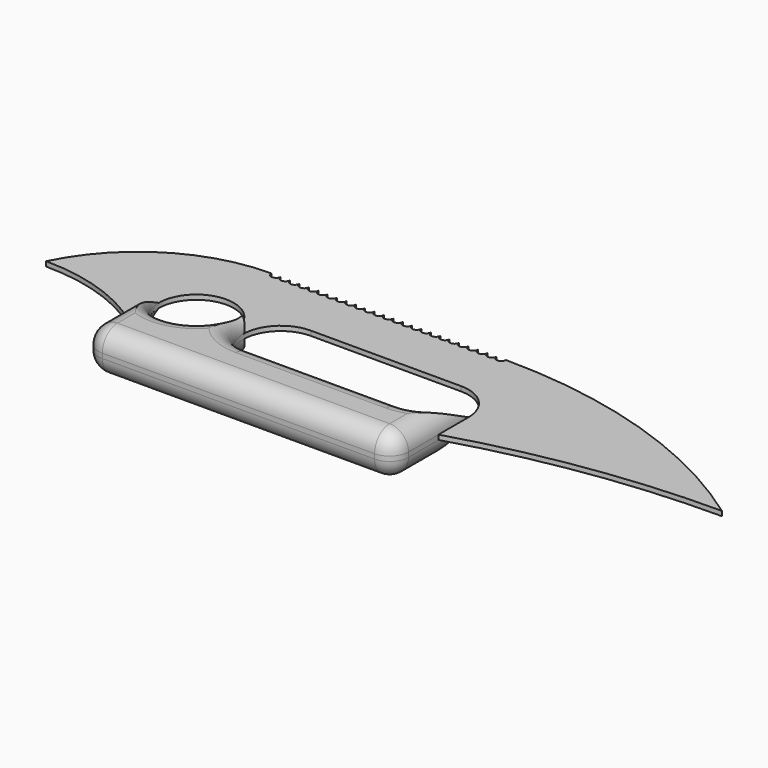
from build123d import *

# Parameters (mm, degrees)
F0_R           = 12.7
F1_DEPTH       = 1.5875
F3_DEPTH       = 6.35
F5_DEPTH       = 6.35
F6_T1_DEPTH    = 92.075
F6_T3_DEPTH    = 41.275
F6_T5_DEPTH    = 50.8
F6_T8_ANGLE    = 323.4698049006
F6_T10_ANGLE   = 90
F6_T12_ANGLE   = 90
F6_T14_ANGLE   = 161.6484946187
F6_T16_ANGLE   = 161.6484946187
F6_2_T1_DEPTH  = 92.075
F6_2_T3_DEPTH  = 41.275
F6_2_T5_DEPTH  = 50.8
F6_2_T8_ANGLE  = 323.4698049006
F6_2_T10_ANGLE = 161.6484946187
F6_2_T12_ANGLE = 90
F6_2_T14_ANGLE = 90
F6_2_T16_ANGLE = 161.6484946187


# Not quite as in the source:
# - a fillet or chamfer that OpenCascade refuses, or shapes differently, is made with other operations: its cross-section is extruded or revolved along the edge and cut away or added


with BuildPart() as f1:
    # F0 (on Top) → F1 (new body)
    with BuildSketch(Plane.XY):
        with BuildLine():
            ThreePointArc((-76.2, -25.4), (-74.3401280605, -29.8901280605), (-69.85, -31.75))
            Line((-69.85, -31.75), (22.225, -31.75))
            ThreePointArc((22.225, -31.75), (26.7151280605, -29.8901280605), (28.575, -25.4))
            Line((28.575, -25.4), (28.575, -12.7))
            ThreePointArc((28.575, -12.7), (70.9696825969, -3.1922325293), (114.3, 0))
            ThreePointArc((114.3, 0), (67.5846294828, 23.6161013967), (15.875, 31.75))
            ThreePointArc((15.875, 31.75), (14.2875, 30.1625), (12.7, 31.75))
            ThreePointArc((12.7, 31.75), (11.1125, 30.1625), (9.525, 31.75))
            ThreePointArc((9.525, 31.75), (7.9375, 30.1625), (6.35, 31.75))
            ThreePointArc((6.35, 31.75), (4.7625, 30.1625), (3.175, 31.75))
            ThreePointArc((3.175, 31.75), (1.5875, 30.1625), (0, 31.75))
            ThreePointArc((0, 31.75), (-1.5875, 30.1625), (-3.175, 31.75))
            ThreePointArc((-3.175, 31.75), (-4.7625, 30.1625), (-6.35, 31.75))
            ThreePointArc((-6.35, 31.75), (-7.9375, 30.1625), (-9.525, 31.75))
            ThreePointArc((-9.525, 31.75), (-11.1125, 30.1625), (-12.7, 31.75))
            ThreePointArc((-12.7, 31.75), (-14.2875, 30.1625), (-15.875, 31.75))
            ThreePointArc((-15.875, 31.75), (-17.4625, 30.1625), (-19.05, 31.75))
            ThreePointArc((-19.05, 31.75), (-20.6375, 30.1625), (-22.225, 31.75))
            ThreePointArc((-22.225, 31.75), (-23.8125, 30.1625), (-25.4, 31.75))
            ThreePointArc((-25.4, 31.75), (-26.9875, 30.1625), (-28.575, 31.75))
            ThreePointArc((-28.575, 31.75), (-30.1625, 30.1625), (-31.75, 31.75))
            ThreePointArc((-31.75, 31.75), (-33.3375, 30.1625), (-34.925, 31.75))
            ThreePointArc((-34.925, 31.75), (-36.5125, 30.1625), (-38.1, 31.75))
            ThreePointArc((-38.1, 31.75), (-39.6875, 30.1625), (-41.275, 31.75))
            ThreePointArc((-41.275, 31.75), (-42.8625, 30.1625), (-44.45, 31.75))
            ThreePointArc((-44.45, 31.75), (-46.0375, 30.1625), (-47.625, 31.75))
            ThreePointArc((-47.625, 31.75), (-49.2125, 30.1625), (-50.8, 31.75))
            ThreePointArc((-50.8, 31.75), (-52.3875, 30.1625), (-53.975, 31.75))
            ThreePointArc((-53.975, 31.75), (-55.5625, 30.1625), (-57.15, 31.75))
            ThreePointArc((-57.15, 31.75), (-58.7375, 30.1625), (-60.325, 31.75))
            ThreePointArc((-60.325, 31.75), (-61.9125, 30.1625), (-63.5, 31.75))
            ThreePointArc((-63.5, 31.75), (-93.4528900943, 23.1596241508), (-114.3, 0))
            ThreePointArc((-114.3, 0), (-94.2195368579, -3.2586105738), (-76.2, -12.7))
            Line((-76.2, -12.7), (-76.2, -25.4))
        make_face()
        with Locations((-63.5, 0)):
            Circle(F0_R, mode=Mode.SUBTRACT)
        with BuildLine():
            Line((15.875, -12.7), (-34.925, -12.7))
            ThreePointArc((-34.925, -12.7), (-47.625, 0), (-34.925, 12.7))
            Line((-34.925, 12.7), (15.875, 12.7))
            ThreePointArc((15.875, 12.7), (28.575, 0), (15.875, -12.7))
        make_face(mode=Mode.SUBTRACT)
    extrude(amount=F1_DEPTH)


with BuildPart() as f3:
    # F2 (on face) → F3 (new body)
    with BuildSketch(Plane.XY.offset(1.5875)):
        with BuildLine():
            Line((-76.2, 0), (-76.2, -12.7))
            Line((-76.2, -12.7), (-76.2, -25.4))
            ThreePointArc((-76.2, -25.4), (-74.3401280605, -29.8901280605), (-69.85, -31.75))
            Line((-69.85, -31.75), (22.225, -31.75))
            ThreePointArc((22.225, -31.75), (26.7151280605, -29.8901280605), (28.575, -25.4))
            Line((28.575, -25.4), (28.575, -12.7))
            Line((28.575, -12.7), (28.575, 0))
            ThreePointArc((28.575, 0), (24.8552561211, -8.9802561211), (15.875, -12.7))
            Line((15.875, -12.7), (-34.925, -12.7))
            ThreePointArc((-34.925, -12.7), (-43.9052561211, -8.9802561211), (-47.625, 0))
            ThreePointArc((-47.625, 0), (-49.2125, 1.5875), (-50.8, 0))
            ThreePointArc((-50.8, 0), (-63.5, -12.7), (-76.2, 0))
        make_face()
    extrude(amount=F3_DEPTH)

    # F6: fillet of radius 6.35 on 8 edges, made by hand

    # F6_s2 → F6_t1 (cut)
    with BuildSketch(Plane.YZ.offset(-69.85)):
        with BuildLine():
            ThreePointArc((-25.4, 7.9375), (-29.8901280605, 6.0776280605), (-31.75, 1.5875))
            Line((-31.75, 1.5875), (-31.75, 7.9375))
            Line((-31.75, 7.9375), (-25.4, 7.9375))
        make_face()
    extrude(amount=F6_T1_DEPTH, mode=Mode.SUBTRACT)

    # F6_s4 → F6_t3 (cut)
    with BuildSketch(Plane.XZ.offset(-15.875)):
        with BuildLine():
            ThreePointArc((-69.85, 7.9375), (-74.3401280605, 6.0776280605), (-76.2, 1.5875))
            Line((-76.2, 1.5875), (-76.2, 7.9375))
            Line((-76.2, 7.9375), (-69.85, 7.9375))
        make_face()
        with BuildLine():
            ThreePointArc((22.225, 7.9375), (26.7151280605, 6.0776280605), (28.575, 1.5875))
            Line((28.575, 1.5875), (28.575, 7.9375))
            Line((28.575, 7.9375), (22.225, 7.9375))
        make_face()
    extrude(amount=F6_T3_DEPTH, mode=Mode.SUBTRACT)

    # F6_s6 → F6_t5 (cut)
    with BuildSketch(Plane.YZ.offset(-34.925)):
        with BuildLine():
            ThreePointArc((-19.05, 7.9375), (-14.5598719395, 6.0776280605), (-12.7, 1.5875))
            Line((-12.7, 1.5875), (-12.7, 7.9375))
            Line((-12.7, 7.9375), (-19.05, 7.9375))
        make_face()
    extrude(amount=F6_T5_DEPTH, mode=Mode.SUBTRACT)

    # F6_s7 → F6_t8 (revolve, cut)
    with BuildSketch(Plane(origin=(-57.2624989836, 18.8990712897, 0), x_dir=(0, 0, 1), z_dir=(-0.949616574, 0.3134140432, 0))):
        with BuildLine():
            ThreePointArc((7.9375, -0.851791742), (6.0776280605, -5.3419198026), (1.5875, -7.201791742))
            Line((1.5875, -7.201791742), (7.9375, -7.201791742))
            Line((7.9375, -7.201791742), (7.9375, -0.851791742))
        make_face()
    revolve(axis=Axis((-63.5, 0, 7.9375), (0, 0, -1)), revolution_arc=F6_T8_ANGLE, mode=Mode.SUBTRACT)

    # F6_s9 → F6_t10 (revolve, cut)
    with BuildSketch(Plane.XZ.offset(25.4)):
        with BuildLine():
            ThreePointArc((-69.85, 7.9375), (-74.3401280605, 6.0776280605), (-76.2, 1.5875))
            Line((-76.2, 1.5875), (-76.2, 7.9375))
            Line((-76.2, 7.9375), (-69.85, 7.9375))
        make_face()
    revolve(axis=Axis((-69.85, -25.4, 7.9375), (0, 0, 1)), revolution_arc=F6_T10_ANGLE, mode=Mode.SUBTRACT)

    # F6_s11 → F6_t12 (revolve, cut)
    with BuildSketch(Plane.YZ.offset(22.225)):
        with BuildLine():
            ThreePointArc((-25.4, 7.9375), (-29.8901280605, 6.0776280605), (-31.75, 1.5875))
            Line((-31.75, 1.5875), (-31.75, 7.9375))
            Line((-31.75, 7.9375), (-25.4, 7.9375))
        make_face()
    revolve(axis=Axis((22.225, -25.4, 7.9375), (0, 0, 1)), revolution_arc=F6_T12_ANGLE, mode=Mode.SUBTRACT)

    # F6_s13 → F6_t14 (revolve, cut)
    with BuildSketch(Plane.YZ.offset(-34.925)):
        with BuildLine():
            ThreePointArc((-19.05, 7.9375), (-14.5598719395, 6.0776280605), (-12.7, 1.5875))
            Line((-12.7, 1.5875), (-12.7, 7.9375))
            Line((-12.7, 7.9375), (-19.05, 7.9375))
        make_face()
    revolve(axis=Axis((-34.925, 0, 7.9375), (0, 0, -1)), revolution_arc=F6_T14_ANGLE, mode=Mode.SUBTRACT)

    # F6_s15 → F6_t16 (revolve, cut)
    with BuildSketch(Plane(origin=(14.3013448994, -4.7439840162, 0), x_dir=(0, 0, 1), z_dir=(-0.9491428342, 0.3148458041, 0))):
        with BuildLine():
            ThreePointArc((7.9375, 24.0481771399), (6.0776280605, 19.5580490793), (1.5875, 17.6981771399))
            Line((1.5875, 17.6981771399), (7.9375, 17.6981771399))
            Line((7.9375, 17.6981771399), (7.9375, 24.0481771399))
        make_face()
    revolve(axis=Axis((15.875, 0, 7.9375), (0, 0, -1)), revolution_arc=F6_T16_ANGLE, mode=Mode.SUBTRACT)


with BuildPart() as f5:
    # F4 (on face) → F5 (new body)
    with BuildSketch(Plane(origin=(0, 0, 0), x_dir=(1, 0, 0), z_dir=(0, 0, -1))):
        with BuildLine():
            Line((28.575, 0), (28.575, 12.7))
            Line((28.575, 12.7), (28.575, 25.4))
            ThreePointArc((28.575, 25.4), (26.7151280605, 29.8901280605), (22.225, 31.75))
            Line((22.225, 31.75), (-69.85, 31.75))
            ThreePointArc((-69.85, 31.75), (-74.3401280605, 29.8901280605), (-76.2, 25.4))
            Line((-76.2, 25.4), (-76.2, 12.7))
            Line((-76.2, 12.7), (-76.2, 0))
            ThreePointArc((-76.2, 0), (-63.5, 12.7), (-50.8, 0))
            ThreePointArc((-50.8, 0), (-49.2125, -1.5875), (-47.625, 0))
            ThreePointArc((-47.625, 0), (-43.9052561211, 8.9802561211), (-34.925, 12.7))
            Line((-34.925, 12.7), (15.875, 12.7))
            ThreePointArc((15.875, 12.7), (24.8552561211, 8.9802561211), (28.575, 0))
        make_face()
    extrude(amount=F5_DEPTH)

    # F6#2: fillet of radius 6.35 on 8 edges, made by hand

    # F6_2_s2 → F6_2_t1 (cut)
    with BuildSketch(Plane.YZ.offset(-69.85)):
        with BuildLine():
            ThreePointArc((-31.75, 0), (-29.8901280605, -4.4901280605), (-25.4, -6.35))
            Line((-25.4, -6.35), (-31.75, -6.35))
            Line((-31.75, -6.35), (-31.75, 0))
        make_face()
    extrude(amount=F6_2_T1_DEPTH, mode=Mode.SUBTRACT)

    # F6_2_s4 → F6_2_t3 (cut)
    with BuildSketch(Plane.XZ.offset(-15.875)):
        with BuildLine():
            ThreePointArc((-76.2, 0), (-74.3401280605, -4.4901280605), (-69.85, -6.35))
            Line((-69.85, -6.35), (-76.2, -6.35))
            Line((-76.2, -6.35), (-76.2, 0))
        make_face()
        with BuildLine():
            ThreePointArc((28.575, 0), (26.7151280605, -4.4901280605), (22.225, -6.35))
            Line((22.225, -6.35), (28.575, -6.35))
            Line((28.575, -6.35), (28.575, 0))
        make_face()
    extrude(amount=F6_2_T3_DEPTH, mode=Mode.SUBTRACT)

    # F6_2_s6 → F6_2_t5 (cut)
    with BuildSketch(Plane.YZ.offset(-34.925)):
        with BuildLine():
            ThreePointArc((-12.7, 0), (-14.5598719395, -4.4901280605), (-19.05, -6.35))
            Line((-19.05, -6.35), (-12.7, -6.35))
            Line((-12.7, -6.35), (-12.7, 0))
        make_face()
    extrude(amount=F6_2_T5_DEPTH, mode=Mode.SUBTRACT)

    # F6_2_s7 → F6_2_t8 (revolve, cut)
    with BuildSketch(Plane(origin=(-57.2624989836, -18.8990712897, 0), x_dir=(0, 0, 1), z_dir=(0.949616574, 0.3134140432, 0))):
        with BuildLine():
            ThreePointArc((0, -32.601791742), (-4.4901280605, -34.4616636815), (-6.35, -38.951791742))
            Line((-6.35, -38.951791742), (-6.35, -32.601791742))
            Line((-6.35, -32.601791742), (0, -32.601791742))
        make_face()
    revolve(axis=Axis((-63.5, 0, -6.35), (0, 0, 1)), revolution_arc=F6_2_T8_ANGLE, mode=Mode.SUBTRACT)

    # F6_2_s9 → F6_2_t10 (revolve, cut)
    with BuildSketch(Plane(origin=(-31.4629587787, -10.4367648357, 0), x_dir=(0, 0, 1), z_dir=(0.9491428342, 0.3148458041, 0))):
        with BuildLine():
            ThreePointArc((0, -23.6959897077), (-4.4901280605, -25.5558616472), (-6.35, -30.0459897077))
            Line((-6.35, -30.0459897077), (-6.35, -23.6959897077))
            Line((-6.35, -23.6959897077), (0, -23.6959897077))
        make_face()
    revolve(axis=Axis((-34.925, 0, -6.35), (0, 0, 1)), revolution_arc=F6_2_T10_ANGLE, mode=Mode.SUBTRACT)

    # F6_2_s11 → F6_2_t12 (revolve, cut)
    with BuildSketch(Plane.YZ.offset(-69.85)):
        with BuildLine():
            ThreePointArc((-31.75, 0), (-29.8901280605, -4.4901280605), (-25.4, -6.35))
            Line((-25.4, -6.35), (-31.75, -6.35))
            Line((-31.75, -6.35), (-31.75, 0))
        make_face()
    revolve(axis=Axis((-69.85, -25.4, -6.35), (0, 0, -1)), revolution_arc=F6_2_T12_ANGLE, mode=Mode.SUBTRACT)

    # F6_2_s13 → F6_2_t14 (revolve, cut)
    with BuildSketch(Plane.XZ.offset(25.4)):
        with BuildLine():
            ThreePointArc((28.575, 0), (26.7151280605, -4.4901280605), (22.225, -6.35))
            Line((22.225, -6.35), (28.575, -6.35))
            Line((28.575, -6.35), (28.575, 0))
        make_face()
    revolve(axis=Axis((22.225, -25.4, -6.35), (0, 0, -1)), revolution_arc=F6_2_T14_ANGLE, mode=Mode.SUBTRACT)

    # F6_2_s15 → F6_2_t16 (revolve, cut)
    with BuildSketch(Plane.YZ.offset(15.875)):
        with BuildLine():
            ThreePointArc((-19.05, -6.35), (-14.5598719395, -4.4901280605), (-12.7, 0))
            Line((-12.7, 0), (-12.7, -6.35))
            Line((-12.7, -6.35), (-19.05, -6.35))
        make_face()
    revolve(axis=Axis((15.875, 0, -6.35), (0, 0, 1)), revolution_arc=F6_2_T16_ANGLE, mode=Mode.SUBTRACT)


solid = Compound([f1.part, f3.part, f5.part])
